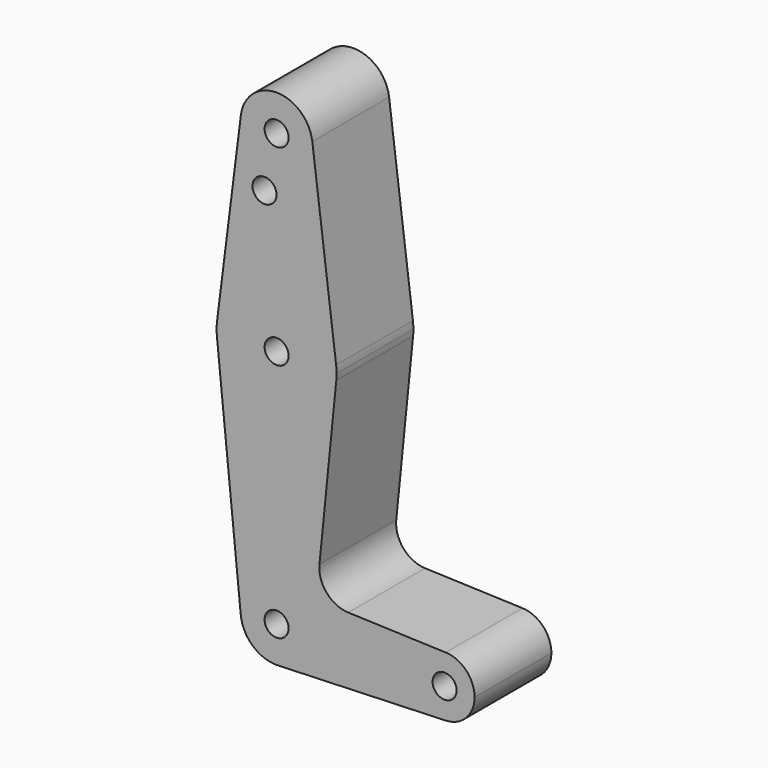
from build123d import *

# Parameters (mm, degrees)
F0_R     = 3.175
F1_DEPTH = 25.4


# Not quite as in the source:
# - a feature names something its author has since deleted; it is built from what else it names


with BuildPart() as f1:
    # F0 (on Front) → F1 (new body)
    with BuildSketch(Plane.XZ):
        with BuildLine():
            ThreePointArc((9.4502929642, 115.490625), (9.5063048942, 114.896483242), (9.525, 114.3))
            ThreePointArc((9.525, 114.3), (-0.596483242, 104.7936951058), (-9.4502929642, 115.490625))
            Line((-9.4502929642, 115.490625), (-15.7504882737, 65.484375))
            ThreePointArc((-15.7504882737, 65.484375), (0, 79.375), (15.7504882737, 65.484375))
            Line((15.7504882737, 65.484375), (9.4502929642, 115.490625))
        make_face()
        with Locations((-3.1970662531, 99.956870079)):
            Circle(F0_R, mode=Mode.SUBTRACT)
        with BuildLine():
            ThreePointArc((15.7954255641, 61.9125), (0, 47.625), (-15.7954255641, 61.9125))
            Line((-15.7954255641, 61.9125), (-9.4772553384, -0.9525))
            ThreePointArc((-9.4772553384, -0.9525), (-0.4768479324, 9.5130563464), (9.525, 0))
            ThreePointArc((9.525, 0), (6.8544082857, -6.6138273378), (0.3401785714, -9.5189234444))
            Line((0.3401785714, -9.5189234444), (44.7334821429, -7.9324362036))
            ThreePointArc((44.7334821429, -7.9324362036), (36.5125, 0), (44.7334821429, 7.9324362036))
            Line((44.7334821429, 7.9324362036), (18.9676000005, 8.8532337108))
            ThreePointArc((18.9676000005, 8.8532337108), (13.2611998974, 11.5713591498), (11.3411865923, 17.5933818124))
            Line((11.3411865923, 17.5933818124), (15.7954255641, 61.9125))
        make_face()
        with BuildLine():
            ThreePointArc((-9.4502929642, 115.490625), (-0.596483242, 104.7936951058), (9.525, 114.3))
            ThreePointArc((9.525, 114.3), (9.5063048942, 114.896483242), (9.4502929642, 115.490625))
            ThreePointArc((9.4502929642, 115.490625), (0, 123.825), (-9.4502929642, 115.490625))
        make_face()
        with Locations((0, 114.3)):
            Circle(F0_R, mode=Mode.SUBTRACT)
        with BuildLine():
            ThreePointArc((15.875, 63.5), (15.8438414904, 64.4941387366), (15.7504882737, 65.484375))
            ThreePointArc((15.7504882737, 65.484375), (0, 79.375), (-15.7504882737, 65.484375))
            ThreePointArc((-15.7504882737, 65.484375), (-15.8737438155, 63.6997054867), (-15.7954255641, 61.9125))
            ThreePointArc((-15.7954255641, 61.9125), (0, 47.625), (15.7954255641, 61.9125))
            ThreePointArc((15.7954255641, 61.9125), (15.8550939106, 62.7052534459), (15.875, 63.5))
        make_face()
        with Locations((0, 63.5)):
            Circle(F0_R, mode=Mode.SUBTRACT)
        with BuildLine():
            ThreePointArc((9.525, 0), (-0.4768479324, 9.5130563464), (-9.4772553384, -0.9525))
            ThreePointArc((-9.4772553384, -0.9525), (-6.2623833816, -7.1769199091), (0.3401785714, -9.5189234444))
            ThreePointArc((0.3401785714, -9.5189234444), (6.8544082857, -6.6138273378), (9.525, 0))
        make_face()
        Circle(F0_R, mode=Mode.SUBTRACT)
        with BuildLine():
            ThreePointArc((44.7334821429, 7.9324362036), (36.5125, 0), (44.7334821429, -7.9324362036))
            ThreePointArc((44.7334821429, -7.9324362036), (50.1620069047, -5.5115227815), (52.3875, 0))
            ThreePointArc((52.3875, 0), (50.1620069047, 5.5115227815), (44.7334821429, 7.9324362036))
        make_face()
        with Locations((44.45, 0)):
            Circle(F0_R, mode=Mode.SUBTRACT)
    extrude(amount=F1_DEPTH)


solid = f1.part
